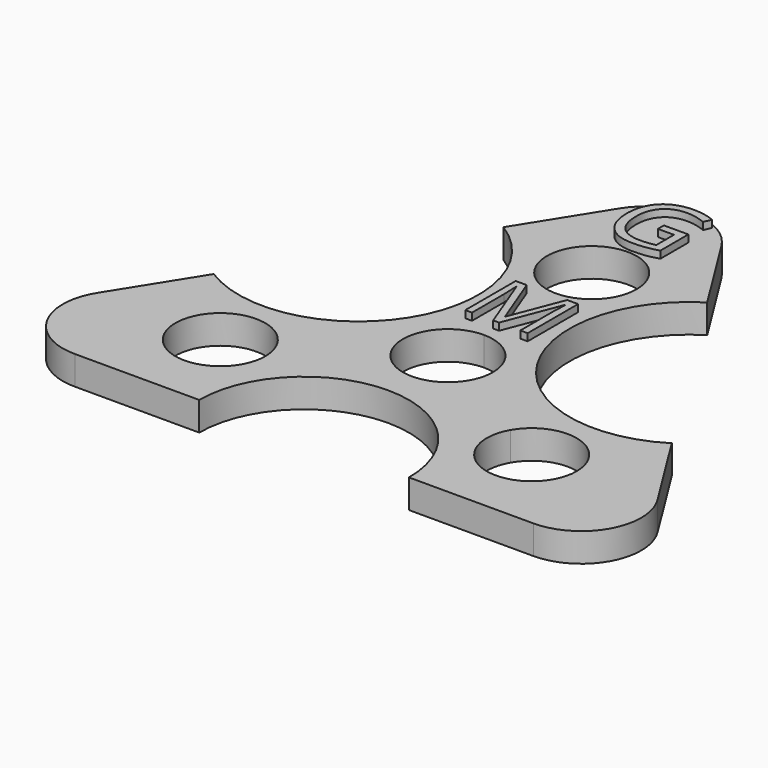
from build123d import *

# Parameters (mm, degrees)
F1_DEPTH       = 6.096
F2_TEXT_SIZE   = 21.3553249422
F2_TEXT_SIZE_2 = 18.7092300993
F3_DEPTH       = 1.524


# Not quite as in the source:
# - Text() gives the source's letters only with a copy of the font that has no kerning and outlines rounded to 1/6400 em; it was checked with that copy


with BuildPart() as f1:
    # F0 (on Top) → F1 (new body)
    with BuildSketch(Plane.XY):
        with BuildLine():
            ThreePointArc((-59.358840651, -18.663363797), (-59.7023695364, -31.5536460827), (-48.5927952922, -38.1))
            Line((-48.5927952922, -38.1), (-22.225, -38.1))
            ThreePointArc((-22.225, -38.1), (0, -15.875), (22.225, -38.1))
            Line((22.225, -38.1), (48.5927952922, -38.1))
            ThreePointArc((48.5927952922, -38.1), (59.7023695364, -31.5536460827), (59.358840651, -18.663363797))
            Line((59.358840651, -18.663363797), (48.5357154109, -1.3665625824))
            ThreePointArc((48.5357154109, -1.3665625824), (13.5303522873, 6.6922557292), (21.5891705989, 41.6976188528))
            Line((21.5891705989, 41.6976188528), (10.7660453588, 58.9944200674))
            ThreePointArc((10.7660453588, 58.9944200674), (0, 64.9577838644), (-10.7660453588, 58.9944200674))
            Line((-10.7660453588, 58.9944200674), (-21.5891705989, 41.6976188528))
            ThreePointArc((-21.5891705989, 41.6976188528), (-13.5303522873, 6.6922557292), (-48.5357154109, -1.3665625824))
            Line((-48.5357154109, -1.3665625824), (-59.358840651, -18.663363797))
        make_face()
        with BuildLine():
            ThreePointArc((-23.4705678842, -19.05), (-42.1960113796, -21.5152514046), (-24.7466759131, -14.2875))
            ThreePointArc((-24.7466759131, -14.2875), (-23.7951243888, -16.5847485954), (-23.4705678842, -19.05))
        make_face(mode=Mode.SUBTRACT)
        with BuildLine():
            ThreePointArc((42.5205678842, -19.05), (30.5303164796, -28.2504434954), (24.7466759131, -14.2875))
            ThreePointArc((24.7466759131, -14.2875), (35.4608192888, -9.8495565046), (42.5205678842, -19.05))
        make_face(mode=Mode.SUBTRACT)
        with BuildLine():
            ThreePointArc((-8.248891971, -4.7625), (-8.248891971, 4.7625), (0, 9.525))
            ThreePointArc((0, 9.525), (6.7351920908, 6.7351920908), (9.525, 0))
            ThreePointArc((9.525, 0), (9.2004434954, -2.4652514046), (8.248891971, -4.7625))
            ThreePointArc((8.248891971, -4.7625), (0, -9.525), (-8.248891971, -4.7625))
        make_face(mode=Mode.SUBTRACT)
        with BuildLine():
            ThreePointArc((0, 28.575), (-6.7351920908, 44.8351920908), (9.525, 38.1))
            ThreePointArc((9.525, 38.1), (6.7351920908, 31.3648079092), (0, 28.575))
        make_face(mode=Mode.SUBTRACT)
    extrude(amount=F1_DEPTH)

    # F2 (on face) → F3 (join)
    with BuildSketch(Plane.XY.offset(6.096)):
        with Locations((-8.2216435637, 48.5033896442)):
            Text('G', F2_TEXT_SIZE, font='Open Sans', text_align=(TextAlign.LEFT, TextAlign.BOTTOM))
        with Locations((-7.9617908498, 12.2534721579)):
            Text('M', F2_TEXT_SIZE_2, font='Open Sans', text_align=(TextAlign.LEFT, TextAlign.BOTTOM))
    extrude(amount=F3_DEPTH)


solid = f1.part
